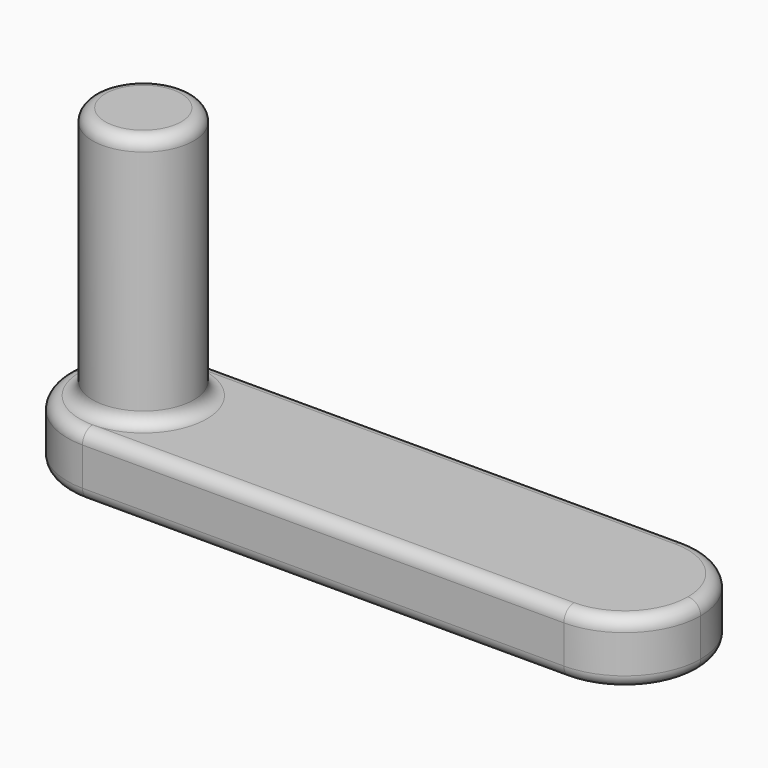
from build123d import *

# Parameters (mm, degrees)
F0_R     = 4
F1_DEPTH = 5
F2_DEPTH = 25
F3_R     = 0.99999


# Not quite as in the source:
# - a fillet or chamfer is up to 0.001 mm smaller than in the source, because OpenCascade refuses the exact size


with BuildPart() as f1:
    # F0 (on Top) → F1 (new body)
    with BuildSketch(Plane.XY):
        with BuildLine():
            ThreePointArc((25, 0), (23.2426406871, 4.2426406871), (19, 6))
            Line((19, 6), (-19, 6))
            ThreePointArc((-19, 6), (-23.2426406871, 4.2426406871), (-25, 0))
            ThreePointArc((-25, 0), (-23.2426406871, -4.2426406871), (-19, -6))
            Line((-19, -6), (19, -6))
            ThreePointArc((19, -6), (23.2426406871, -4.2426406871), (25, 0))
        make_face()
        with Locations((-19, 0)):
            Circle(F0_R, mode=Mode.SUBTRACT)
        with Locations((19, 0)):
            Circle(F0_R, mode=Mode.SUBTRACT)
        with Locations((-19, 0)):
            Circle(F0_R)
        with Locations((19, 0)):
            Circle(F0_R)
    extrude(amount=F1_DEPTH)

    # F0 (on Top) → F2 (join)
    with BuildSketch(Plane.XY):
        with Locations((-19, 0)):
            Circle(F0_R)
    extrude(amount=F2_DEPTH)

    # F3 (radius 1 in the source; OpenCascade refuses exactly that, so slightly less here)
    f3_edges = [f1.edges().sort_by_distance(p)[0] for p in [
        (0, 6, 5),
        (0, 6, 0),
        (-23, 0, 5),
        (-23, 0, 25),
    ]]
    fillet(f3_edges, radius=F3_R)


solid = f1.part
